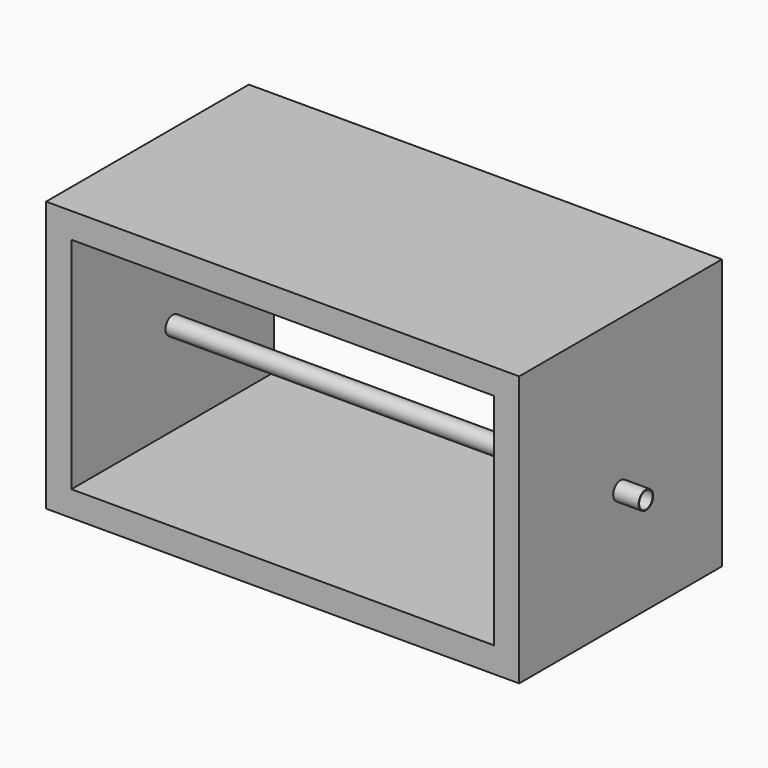
from build123d import *

# Parameters (mm, degrees)
F0_W      = 355.6
F0_H      = 203.2
F0_W_2    = 317.5
F0_H_2    = 165.1
F1_DEPTH  = 95.25
F2_R      = 6.35
F3_DEPTH  = 355.601
F4_R      = 50.8
F4_R_2    = 6.35
F5_DEPTH  = 19.05
F6_R      = 6.35
F7_DEPTH  = 19.05
F9_R      = 6.879532365
F9_R_2    = 6.35
F10_DEPTH = 355.6


# Not quite as in the source:
# - the program builds the solid bodies; features that only make, move or delete a surface that nothing else refers to are left out


with BuildPart() as f1:
    # F0 (on Front) → F1 (new body, symmetric)
    with BuildSketch(Plane.XZ):
        Rectangle(F0_W, F0_H)
        Rectangle(F0_W_2, F0_H_2, mode=Mode.SUBTRACT)
    extrude(amount=F1_DEPTH, both=True)

    # F2 (on face) → F3 (cut, through all)
    with BuildSketch(Plane(origin=(-177.8, 0, 0), x_dir=(0, -1, 0), z_dir=(-1, 0, 0))):
        with Locations((0, -12.7)):
            Circle(F2_R)
    extrude(amount=-F3_DEPTH, mode=Mode.SUBTRACT)


with BuildPart() as f5:
    # F4 (on face) → F5 (new body)
    with BuildSketch(Plane(origin=(-177.8, 0, 0), x_dir=(0, -1, 0), z_dir=(-1, 0, 0))):
        with Locations((0, -12.7)):
            Circle(F4_R)
        with Locations((0, -12.7)):
            Circle(F4_R_2, mode=Mode.SUBTRACT)
    extrude(amount=F5_DEPTH)

    # F6 (on face) → F7 (cut, through all)
    with BuildSketch(Plane(origin=(-196.85, 0, 0), x_dir=(0, -1, 0), z_dir=(-1, 0, 0))):
        with Locations((0, 25.4)):
            Circle(F6_R)
    extrude(amount=-F7_DEPTH, mode=Mode.SUBTRACT)


with BuildPart() as f10:
    # F9 (on face) → F10 (new body)
    with BuildSketch(Plane.YZ.offset(-158.75)):
        with Locations((0, -12.7)):
            Circle(F9_R)
        with Locations((0, -12.7)):
            Circle(F9_R_2, mode=Mode.SUBTRACT)
    extrude(amount=F10_DEPTH)


solid = Compound([f1.part, f5.part, f10.part])
